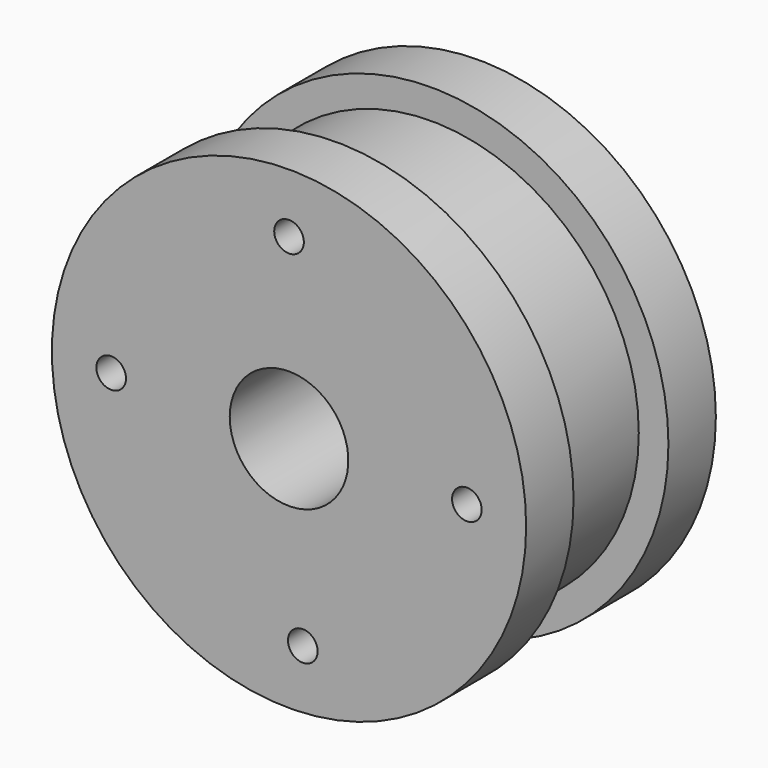
from build123d import *

# Parameters (mm, degrees)
F0_R      = 25.4
F1_DEPTH  = 6.35
F2_R      = 22.225
F3_DEPTH  = 12.7
F4_R      = 25.4
F5_DEPTH  = 6.35
F6_R      = 1.5875
F6_R_2    = 6.35
F7_DEPTH  = 89
F9_D      = 12.7
F11_D     = 3.175
F11_DEPTH = 6.35
F11_TIP   = 0.9538662327
F13_D     = 3.175
F13_DEPTH = 6.35
F13_TIP   = 0.9538662327
F15_D     = 3.175
F15_DEPTH = 6.35
F15_TIP   = 0.9538662327
F17_D     = 3.175
F17_DEPTH = 6.35
F17_TIP   = 0.9538662327


# Not quite as in the source:
# - an extrude ends at something that could not be found from the text; its depth is read off the source's solid


with BuildPart() as f1:
    # F0 (on Front) → F1 (new body)
    with BuildSketch(Plane.XZ):
        Circle(F0_R)
    extrude(amount=F1_DEPTH)

    # F2 (on face) → F3 (join)
    with BuildSketch(Plane.XZ.offset(6.35)):
        Circle(F2_R)
    extrude(amount=F3_DEPTH)

    # F4 (on face) → F5 (join)
    with BuildSketch(Plane.XZ.offset(19.05)):
        Circle(F4_R)
    extrude(amount=F5_DEPTH)

    # F6 (on face) → F7 (cut, through all)
    with BuildSketch(Plane.XZ.offset(25.4)):
        with Locations((0, -20.6375)):
            Circle(F6_R)
        with Locations((20.6375, 0)):
            Circle(F6_R)
        with Locations((0, 20.6375)):
            Circle(F6_R)
        with Locations((-20.6375, 0)):
            Circle(F6_R)
        Circle(F6_R_2)
    extrude(amount=F7_DEPTH, mode=Mode.SUBTRACT)

    # F9 (through all)
    with Locations(Plane.XZ.offset(25.4)):
        with Locations((0, 0)):
            Hole(F9_D / 2)

    # F11
    with Locations(Plane.XZ.offset(25.4)):
        with Locations((19.05, 0)):
            Hole(F11_D / 2, depth=F11_DEPTH)
            with Locations((0, 0, -(F11_DEPTH + F11_TIP / 2))):  # 118° drill point
                Cone(0, F11_D / 2, F11_TIP, mode=Mode.SUBTRACT)

    # F13
    with Locations(Plane.XZ.offset(25.4)):
        with Locations((0, 19.05)):
            Hole(F13_D / 2, depth=F13_DEPTH)
            with Locations((0, 0, -(F13_DEPTH + F13_TIP / 2))):  # 118° drill point
                Cone(0, F13_D / 2, F13_TIP, mode=Mode.SUBTRACT)

    # F15
    with Locations(Plane.XZ.offset(25.4)):
        with Locations((-19.05, 0)):
            Hole(F15_D / 2, depth=F15_DEPTH)
            with Locations((0, 0, -(F15_DEPTH + F15_TIP / 2))):  # 118° drill point
                Cone(0, F15_D / 2, F15_TIP, mode=Mode.SUBTRACT)

    # F17
    with Locations(Plane.XZ.offset(25.4)):
        with Locations((1.4731416013, -19.0587695688)):
            Hole(F17_D / 2, depth=F17_DEPTH)
            with Locations((0, 0, -(F17_DEPTH + F17_TIP / 2))):  # 118° drill point
                Cone(0, F17_D / 2, F17_TIP, mode=Mode.SUBTRACT)


solid = f1.part
